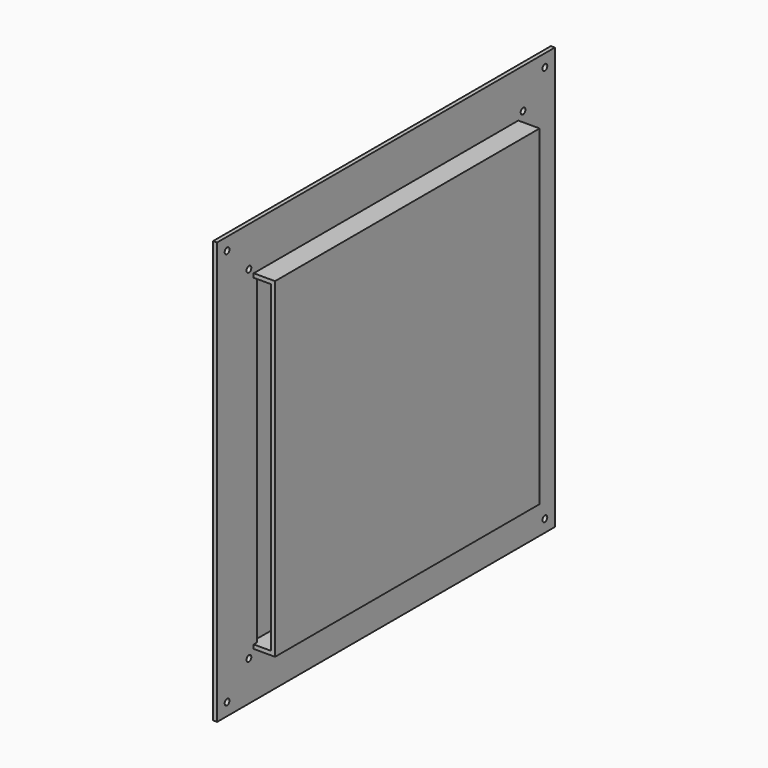
from build123d import *

# Parameters (mm, degrees)
F0_W        = 170
F0_H        = 170
F0_W_2      = 133.2
F0_H_2      = 133.2
F1_DEPTH    = 1.6
F2_DEPTH    = 10.2
F3_T        = 1.6
F3_T3_DEPTH = 136.4
F3_T5_DEPTH = 136.4
F4_W        = 7
F4_H        = 130
F5_DEPTH    = 1.6
F6_D        = 2.4
F7_W        = 148
F7_H        = 148
F7_R        = 2
F8_DEPTH    = 1.6


# Not quite as in the source:
# - a shell that OpenCascade refuses in one call is made with other operations: the cavity is built on its own and cut out


with BuildPart() as f1:
    # F0 (on Right) → F1 (new body)
    with BuildSketch(Plane.YZ):
        Rectangle(F0_W, F0_H)
        Rectangle(F0_W_2, F0_H_2, mode=Mode.SUBTRACT)
    extrude(amount=F1_DEPTH)

    # F0 (on Right) → F2 (join)
    with BuildSketch(Plane.YZ):
        Rectangle(F0_W_2, F0_H_2)
    extrude(amount=F2_DEPTH)

    # F3: shell of thickness 1.6, made by hand


with BuildPart() as f3_core1:
    # F3_t2: copy of F1
    add(f1.part)

    # the walls: a layer under each face that stays
    f3_faces = [f3_core1.faces().sort_by_distance(p)[0] for p in [
        (0.8, 0, -85),
        (0.8, -85, 0),
        (0.8, 85, 0),
        (1.6, -72.8571428571, -72.8571428571),
        (0.8, 0, 85),
        (5.9, 66.6, 0),
        (5.9, 0, -66.6),
        (5.9, -66.6, 0),
        (5.9, 0, 66.6),
        (10.2, 0, 0),
    ]]
    thicken(f3_faces, amount=-F3_T, mode=Mode.SUBTRACT)

    # F3_s4 → F3_t3 (cut)
    with BuildSketch(Plane.XY.offset(-68.2)):
        Polygon((1.616, 66.616), (0, 66.6), (0, 65), (1.6, 65), align=None)
        Polygon((1.616, -66.616), (0, -66.6), (0, -65), (1.6, -65), align=None)
    extrude(amount=F3_T3_DEPTH, mode=Mode.SUBTRACT)

    # F3_s6 → F3_t5 (cut)
    with BuildSketch(Plane.XZ.offset(-68.2)):
        Polygon((1.616, -66.616), (0, -66.6), (0, -65), (1.6, -65), align=None)
        Polygon((1.616, 66.616), (0, 66.6), (0, 65), (1.6, 65), align=None)
    extrude(amount=F3_T5_DEPTH, mode=Mode.SUBTRACT)


with BuildPart() as f1_1:
    add(f1.part)

    # what is left inside the walls is the cavity
    f3_cavity = [f3_core1.part.solids().sort_by_distance(p)[0] for p in [
        (0.016, 0, -21.666667),
    ]]
    add(f3_cavity, mode=Mode.SUBTRACT)

    # F4 (on face) → F5 (cut, through all)
    with BuildSketch(Plane.XZ.offset(66.6)):
        with Locations((5.1, 0)):
            Rectangle(F4_W, F4_H)
    extrude(amount=-F5_DEPTH, mode=Mode.SUBTRACT)

    # F6 (through all)
    with Locations(Plane(origin=(0, 0, 0), x_dir=(0, 1, 0), z_dir=(-1, 0, 0))):
        with Locations((80, -80), (69, -69), (69, 69), (80, 80), (-69, 69), (-80, 80), (-80, -80), (-69, -69)):
            Hole(F6_D / 2)


with BuildPart() as f8:
    # F7 (on face) → F8 (new body)
    with BuildSketch(Plane.YZ):
        Rectangle(F7_W, F7_H)
        with Locations((-69, -69)):
            Circle(F7_R, mode=Mode.SUBTRACT)
        with Locations((69, -69)):
            Circle(F7_R, mode=Mode.SUBTRACT)
        with Locations((-69, 69)):
            Circle(F7_R, mode=Mode.SUBTRACT)
        with Locations((69, 69)):
            Circle(F7_R, mode=Mode.SUBTRACT)
    extrude(amount=-F8_DEPTH)


solid = Compound([f1_1.part, f8.part])
